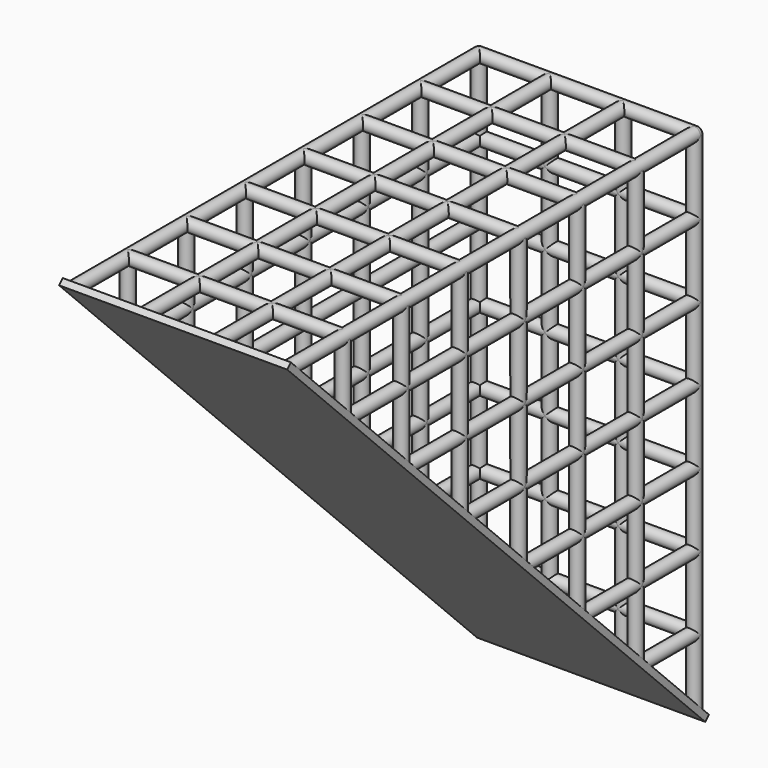
from build123d import *

# Parameters (mm, degrees)
F5_R      = 0.3
F6_DEPTH  = 10
F7_R      = 0.3
F8_DEPTH  = 23.8
F9_R      = 0.3
F10_DEPTH = 23.8
F25_W     = 10.6
F25_H     = 34.346151
F26_DEPTH = 0.3
F27_W     = 18
F27_H     = 42.84
F28_DEPTH = 25


with BuildPart() as f6:
    # F5 (on Right) → F6 (new body)
    with BuildSketch(Plane.YZ):
        Circle(F5_R)
    extrude(amount=F6_DEPTH)


with BuildPart() as f6b:
    # F5 (on Right) → F6, piece 2 (new body)
    with BuildSketch(Plane.YZ):
        with Locations((3.4, 0)):
            Circle(F5_R)
    extrude(amount=F6_DEPTH)


with BuildPart() as f6c:
    # F5 (on Right) → F6, piece 3 (new body)
    with BuildSketch(Plane.YZ):
        with Locations((6.8, 0)):
            Circle(F5_R)
    extrude(amount=F6_DEPTH)


with BuildPart() as f6d:
    # F5 (on Right) → F6, piece 4 (new body)
    with BuildSketch(Plane.YZ):
        with Locations((10.2, 0)):
            Circle(F5_R)
    extrude(amount=F6_DEPTH)


with BuildPart() as f6e:
    # F5 (on Right) → F6, piece 5 (new body)
    with BuildSketch(Plane.YZ):
        with Locations((13.6, 0)):
            Circle(F5_R)
    extrude(amount=F6_DEPTH)


with BuildPart() as f6f:
    # F5 (on Right) → F6, piece 6 (new body)
    with BuildSketch(Plane.YZ):
        with Locations((17, 0)):
            Circle(F5_R)
    extrude(amount=F6_DEPTH)


with BuildPart() as f6g:
    # F5 (on Right) → F6, piece 7 (new body)
    with BuildSketch(Plane.YZ):
        with Locations((20.4, 0)):
            Circle(F5_R)
    extrude(amount=F6_DEPTH)


with BuildPart() as f6h:
    # F5 (on Right) → F6, piece 8 (new body)
    with BuildSketch(Plane.YZ):
        with Locations((23.8, 0)):
            Circle(F5_R)
    extrude(amount=F6_DEPTH)


with BuildPart() as f6i:
    # F5 (on Right) → F6, piece 9 (new body)
    with BuildSketch(Plane.YZ):
        with Locations((23.8, -3.4)):
            Circle(F5_R)
    extrude(amount=F6_DEPTH)


with BuildPart() as f6j:
    # F5 (on Right) → F6, piece 10 (new body)
    with BuildSketch(Plane.YZ):
        with Locations((23.8, -6.8)):
            Circle(F5_R)
    extrude(amount=F6_DEPTH)


with BuildPart() as f6k:
    # F5 (on Right) → F6, piece 11 (new body)
    with BuildSketch(Plane.YZ):
        with Locations((23.8, -10.2)):
            Circle(F5_R)
    extrude(amount=F6_DEPTH)


with BuildPart() as f6l:
    # F5 (on Right) → F6, piece 12 (new body)
    with BuildSketch(Plane.YZ):
        with Locations((23.8, -13.6)):
            Circle(F5_R)
    extrude(amount=F6_DEPTH)


with BuildPart() as f6m:
    # F5 (on Right) → F6, piece 13 (new body)
    with BuildSketch(Plane.YZ):
        with Locations((23.8, -17)):
            Circle(F5_R)
    extrude(amount=F6_DEPTH)


with BuildPart() as f6n:
    # F5 (on Right) → F6, piece 14 (new body)
    with BuildSketch(Plane.YZ):
        with Locations((23.8, -20.4)):
            Circle(F5_R)
    extrude(amount=F6_DEPTH)


with BuildPart() as f6o:
    # F5 (on Right) → F6, piece 15 (new body)
    with BuildSketch(Plane.YZ):
        with Locations((23.8, -23.8)):
            Circle(F5_R)
    extrude(amount=F6_DEPTH)


with BuildPart() as f8:
    # F7 (on offset) → F8 (new body)
    with BuildSketch(Plane.XY):
        Circle(F7_R)
    extrude(amount=-F8_DEPTH)


with BuildPart() as f8b:
    # F7 (on offset) → F8, piece 2 (new body)
    with BuildSketch(Plane.XY):
        with Locations((0, 3.4)):
            Circle(F7_R)
    extrude(amount=-F8_DEPTH)


with BuildPart() as f8c:
    # F7 (on offset) → F8, piece 3 (new body)
    with BuildSketch(Plane.XY):
        with Locations((0, 6.8)):
            Circle(F7_R)
    extrude(amount=-F8_DEPTH)


with BuildPart() as f8d:
    # F7 (on offset) → F8, piece 4 (new body)
    with BuildSketch(Plane.XY):
        with Locations((0, 10.2)):
            Circle(F7_R)
    extrude(amount=-F8_DEPTH)


with BuildPart() as f8e:
    # F7 (on offset) → F8, piece 5 (new body)
    with BuildSketch(Plane.XY):
        with Locations((0, 13.6)):
            Circle(F7_R)
    extrude(amount=-F8_DEPTH)


with BuildPart() as f8f:
    # F7 (on offset) → F8, piece 6 (new body)
    with BuildSketch(Plane.XY):
        with Locations((0, 17)):
            Circle(F7_R)
    extrude(amount=-F8_DEPTH)


with BuildPart() as f8g:
    # F7 (on offset) → F8, piece 7 (new body)
    with BuildSketch(Plane.XY):
        with Locations((0, 20.4)):
            Circle(F7_R)
    extrude(amount=-F8_DEPTH)


with BuildPart() as f8h:
    # F7 (on offset) → F8, piece 8 (new body)
    with BuildSketch(Plane.XY):
        with Locations((0, 23.8)):
            Circle(F7_R)
    extrude(amount=-F8_DEPTH)


with BuildPart() as f8i:
    # F7 (on offset) → F8, piece 9 (new body)
    with BuildSketch(Plane.XY):
        with Locations((10, 0)):
            Circle(F7_R)
    extrude(amount=-F8_DEPTH)


with BuildPart() as f8j:
    # F7 (on offset) → F8, piece 10 (new body)
    with BuildSketch(Plane.XY):
        with Locations((10, 3.4)):
            Circle(F7_R)
    extrude(amount=-F8_DEPTH)


with BuildPart() as f8k:
    # F7 (on offset) → F8, piece 11 (new body)
    with BuildSketch(Plane.XY):
        with Locations((10, 6.8)):
            Circle(F7_R)
    extrude(amount=-F8_DEPTH)


with BuildPart() as f8l:
    # F7 (on offset) → F8, piece 12 (new body)
    with BuildSketch(Plane.XY):
        with Locations((10, 10.2)):
            Circle(F7_R)
    extrude(amount=-F8_DEPTH)


with BuildPart() as f8m:
    # F7 (on offset) → F8, piece 13 (new body)
    with BuildSketch(Plane.XY):
        with Locations((10, 13.6)):
            Circle(F7_R)
    extrude(amount=-F8_DEPTH)


with BuildPart() as f8n:
    # F7 (on offset) → F8, piece 14 (new body)
    with BuildSketch(Plane.XY):
        with Locations((10, 17)):
            Circle(F7_R)
    extrude(amount=-F8_DEPTH)


with BuildPart() as f8o:
    # F7 (on offset) → F8, piece 15 (new body)
    with BuildSketch(Plane.XY):
        with Locations((10, 20.4)):
            Circle(F7_R)
    extrude(amount=-F8_DEPTH)


with BuildPart() as f8p:
    # F7 (on offset) → F8, piece 16 (new body)
    with BuildSketch(Plane.XY):
        with Locations((3.3, 23.8)):
            Circle(F7_R)
    extrude(amount=-F8_DEPTH)


with BuildPart() as f8q:
    # F7 (on offset) → F8, piece 17 (new body)
    with BuildSketch(Plane.XY):
        with Locations((6.7, 23.8)):
            Circle(F7_R)
    extrude(amount=-F8_DEPTH)


with BuildPart() as f8r:
    # F7 (on offset) → F8, piece 18 (new body)
    with BuildSketch(Plane.XY):
        with Locations((10, 23.8)):
            Circle(F7_R)
    extrude(amount=-F8_DEPTH)


with BuildPart() as f10:
    # F9 (on offset) → F10 (new body)
    with BuildSketch(Plane.XZ):
        with Locations((0, -23.8)):
            Circle(F9_R)
    extrude(amount=-F10_DEPTH)


with BuildPart() as f10b:
    # F9 (on offset) → F10, piece 2 (new body)
    with BuildSketch(Plane.XZ):
        with Locations((0, -20.4)):
            Circle(F9_R)
    extrude(amount=-F10_DEPTH)


with BuildPart() as f10c:
    # F9 (on offset) → F10, piece 3 (new body)
    with BuildSketch(Plane.XZ):
        with Locations((0, -17)):
            Circle(F9_R)
    extrude(amount=-F10_DEPTH)


with BuildPart() as f10d:
    # F9 (on offset) → F10, piece 4 (new body)
    with BuildSketch(Plane.XZ):
        with Locations((0, -13.6)):
            Circle(F9_R)
    extrude(amount=-F10_DEPTH)


with BuildPart() as f10e:
    # F9 (on offset) → F10, piece 5 (new body)
    with BuildSketch(Plane.XZ):
        with Locations((0, -10.2)):
            Circle(F9_R)
    extrude(amount=-F10_DEPTH)


with BuildPart() as f10f:
    # F9 (on offset) → F10, piece 6 (new body)
    with BuildSketch(Plane.XZ):
        with Locations((0, -6.8)):
            Circle(F9_R)
    extrude(amount=-F10_DEPTH)


with BuildPart() as f10g:
    # F9 (on offset) → F10, piece 7 (new body)
    with BuildSketch(Plane.XZ):
        with Locations((0, -3.4)):
            Circle(F9_R)
    extrude(amount=-F10_DEPTH)


with BuildPart() as f10h:
    # F9 (on offset) → F10, piece 8 (new body)
    with BuildSketch(Plane.XZ):
        Circle(F9_R)
    extrude(amount=-F10_DEPTH)


with BuildPart() as f10i:
    # F9 (on offset) → F10, piece 9 (new body)
    with BuildSketch(Plane.XZ):
        with Locations((10, -23.8)):
            Circle(F9_R)
    extrude(amount=-F10_DEPTH)


with BuildPart() as f10j:
    # F9 (on offset) → F10, piece 10 (new body)
    with BuildSketch(Plane.XZ):
        with Locations((10, -20.4)):
            Circle(F9_R)
    extrude(amount=-F10_DEPTH)


with BuildPart() as f10k:
    # F9 (on offset) → F10, piece 11 (new body)
    with BuildSketch(Plane.XZ):
        with Locations((10, -17)):
            Circle(F9_R)
    extrude(amount=-F10_DEPTH)


with BuildPart() as f10l:
    # F9 (on offset) → F10, piece 12 (new body)
    with BuildSketch(Plane.XZ):
        with Locations((10, -13.6)):
            Circle(F9_R)
    extrude(amount=-F10_DEPTH)


with BuildPart() as f10m:
    # F9 (on offset) → F10, piece 13 (new body)
    with BuildSketch(Plane.XZ):
        with Locations((10, -10.2)):
            Circle(F9_R)
    extrude(amount=-F10_DEPTH)


with BuildPart() as f10n:
    # F9 (on offset) → F10, piece 14 (new body)
    with BuildSketch(Plane.XZ):
        with Locations((10, -6.8)):
            Circle(F9_R)
    extrude(amount=-F10_DEPTH)


with BuildPart() as f10o:
    # F9 (on offset) → F10, piece 15 (new body)
    with BuildSketch(Plane.XZ):
        with Locations((10, -3.4)):
            Circle(F9_R)
    extrude(amount=-F10_DEPTH)


with BuildPart() as f10p:
    # F9 (on offset) → F10, piece 16 (new body)
    with BuildSketch(Plane.XZ):
        with Locations((3.3, 0)):
            Circle(F9_R)
    extrude(amount=-F10_DEPTH)


with BuildPart() as f10q:
    # F9 (on offset) → F10, piece 17 (new body)
    with BuildSketch(Plane.XZ):
        with Locations((6.7, 0)):
            Circle(F9_R)
    extrude(amount=-F10_DEPTH)


with BuildPart() as f10r:
    # F9 (on offset) → F10, piece 18 (new body)
    with BuildSketch(Plane.XZ):
        with Locations((10, 0)):
            Circle(F9_R)
    extrude(amount=-F10_DEPTH)


with BuildPart() as f6g_1:
    add(f6g.part)

    # F11: union F6f, F6e, F6i, F6d, F6c, F6j, F6k, F6l, F6m, F6n, F6o, F6b, F8r, F8q, F8p, F8o, F8n, F8m, F8l, F6, F8, F8k, F8i, F8j, F8g, F8h, F8f, F8e, F8d, F8c, F6h, F8b, F10, F10b, F10c, F10d, F10e, F10f, F10g, F10h, F10i, F10j, F10k, F10l, F10m, F10n, F10o, F10p, F10q, F10r
    add(f6f.part)
    add(f6e.part)
    add(f6i.part)
    add(f6d.part)
    add(f6c.part)
    add(f6j.part)
    add(f6k.part)
    add(f6l.part)
    add(f6m.part)
    add(f6n.part)
    add(f6o.part)
    add(f6b.part)
    add(f8r.part)
    add(f8q.part)
    add(f8p.part)
    add(f8o.part)
    add(f8n.part)
    add(f8m.part)
    add(f8l.part)
    add(f6.part)
    add(f8.part)
    add(f8k.part)
    add(f8i.part)
    add(f8j.part)
    add(f8g.part)
    add(f8h.part)
    add(f8f.part)
    add(f8e.part)
    add(f8d.part)
    add(f8c.part)
    add(f6h.part)
    add(f8b.part)
    add(f10.part)
    add(f10b.part)
    add(f10c.part)
    add(f10d.part)
    add(f10e.part)
    add(f10f.part)
    add(f10g.part)
    add(f10h.part)
    add(f10i.part)
    add(f10j.part)
    add(f10k.part)
    add(f10l.part)
    add(f10m.part)
    add(f10n.part)
    add(f10o.part)
    add(f10p.part)
    add(f10q.part)
    add(f10r.part)

    # F13 (on face) → F14 (revolve)
    with BuildSketch(Plane.XY):
        with BuildLine():
            Line((10.3, 0), (10, 0))
            Line((10, 0), (10, -0.3))
            ThreePointArc((10, -0.3), (10.212132, -0.212132), (10.3, 0))
        make_face()
    revolve(axis=Axis((10, -0.191384, 0), (0, -1, 0)))

    # F12 (on face) → F15 (revolve)
    with BuildSketch(Plane.XY):
        with BuildLine():
            Line((10, 24.1), (10, 23.8))
            Line((10, 23.8), (10.3, 23.8))
            ThreePointArc((10.3, 23.8), (10.212132, 24.012132), (10, 24.1))
        make_face()
    revolve(axis=Axis((10, 24.076715, 0), (0, 1, 0)))

    # F6_face (on face) → F17 (revolve)
    with BuildSketch(Plane(origin=(0, 23.927324, 0.127324), x_dir=(0, 1, 0), z_dir=(-1, 0, 0))):
        with BuildLine():
            Line((0.172676, 0.127324), (-0.127324, 0.127324))
            Line((-0.127324, 0.127324), (-0.127324, -0.172676))
            ThreePointArc((-0.127324, -0.172676), (0.084808, -0.084808), (0.172676, 0.127324))
        make_face()
    revolve(axis=Axis((0, 24.193682, 0), (0, 1, 0)))

    # F8_face1 (on face) → F19 (revolve)
    with BuildSketch(Plane(origin=(10.127324, 23.927324, -23.8), x_dir=(1, 0, 0), z_dir=(0, 0, -1))):
        with BuildLine():
            Line((0.172676, 0.127324), (-0.127324, 0.127324))
            Line((-0.127324, 0.127324), (-0.127324, -0.172676))
            ThreePointArc((-0.127324, -0.172676), (0.084808, -0.084808), (0.172676, 0.127324))
        make_face()
    revolve(axis=Axis((5.266674, 23.8, -23.8), (1, 0, 0)))

    # F8_face1 (on face) → F20 (revolve)
    with BuildSketch(Plane(origin=(10.127324, 23.927324, -23.8), x_dir=(1, 0, 0), z_dir=(0, 0, -1))):
        with BuildLine():
            Line((-10.127324, -0.172676), (-10.127324, 0.127324))
            Line((-10.127324, 0.127324), (-10.427324, 0.127324))
            ThreePointArc((-10.427324, 0.127324), (-10.339456, -0.084808), (-10.127324, -0.172676))
        make_face()
    revolve(axis=Axis((-0.15, 23.8, -23.8), (1, 0, 0)))

    # F21 (on face) → F22 (revolve)
    with BuildSketch(Plane(origin=(0, 0, 0), x_dir=(0, -1, 0), z_dir=(-1, 0, 0))):
        with BuildLine():
            Line((0, 0.3), (0, 0))
            Line((0, 0), (0.3, 0))
            ThreePointArc((0.3, 0), (0.212132, 0.212132), (0, 0.3))
        make_face()
    revolve(axis=Axis((0, -0.242, 0), (0, -1, 0)))

    # F25 (on line) → F26 (join)
    with BuildSketch(Plane(origin=(0, 0, 0), x_dir=(-1, 0, 0), z_dir=(0, 0.707107, 0.707107))):
        with Locations((-5, -16.873076)):
            Rectangle(F25_W, F25_H)
    extrude(amount=F26_DEPTH)

    # F27 (on line) → F28 (cut)
    with BuildSketch(Plane(origin=(0, 0, 0), x_dir=(-1, 0, 0), z_dir=(0, 0.707107, 0.707107))):
        with Locations((-5, -17.42)):
            Rectangle(F27_W, F27_H)
    extrude(amount=-F28_DEPTH, mode=Mode.SUBTRACT)


solid = f6g_1.part
